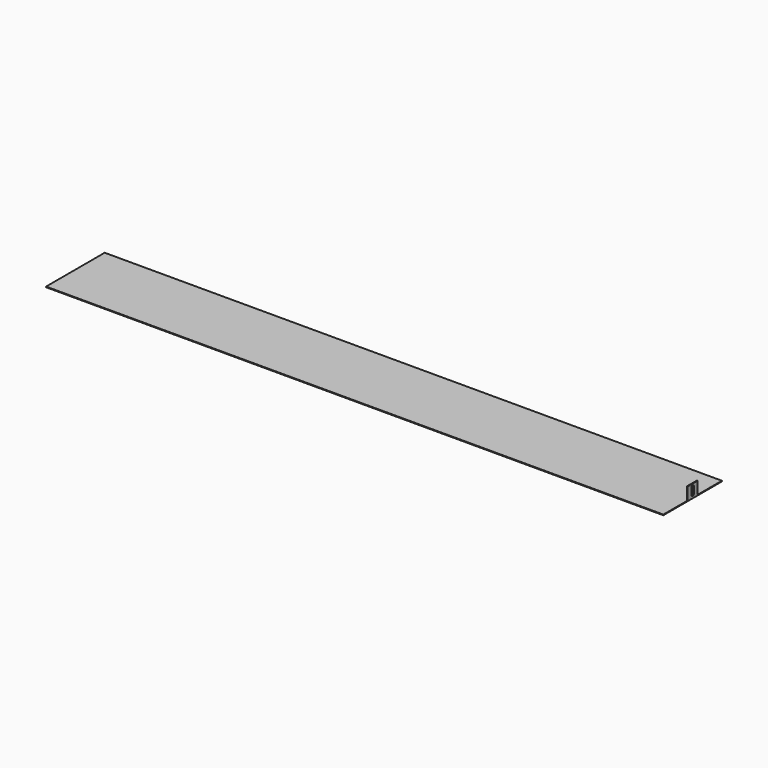
from build123d import *

# Parameters (mm, degrees)
F0_W     = 1500
F0_H     = 178
F1_DEPTH = 1.5875
F2_W     = 30
F2_H     = 30
F3_DEPTH = 1.5875


# Not quite as in the source:
# - a length typed as a fraction of an inch, garbled in the dataset ("3 / 203.2 mm" for 3/8 in), is restored


with BuildPart() as f1:
    # F0 (on Top) → F1 (new body)
    with BuildSketch(Plane.XY):
        with Locations((673.9510029554, 75.5837445271)):
            Rectangle(F0_W, F0_H)
    extrude(amount=F1_DEPTH)

    # F2 (on face) → F3 (join)
    with BuildSketch(Plane.YZ.offset(1423.9510029554)):
        with Locations((75.5837445271, 16.5875)):
            Rectangle(F2_W, F2_H)
        with BuildLine():
            ThreePointArc((71.5837445271, 24.0875), (75.5837445271, 28.0875), (79.5837445271, 24.0875))
            Line((79.5837445271, 24.0875), (79.5837445271, 9.0875))
            ThreePointArc((79.5837445271, 9.0875), (75.5837445271, 5.0875), (71.5837445271, 9.0875))
            Line((71.5837445271, 9.0875), (71.5837445271, 24.0875))
        make_face(mode=Mode.SUBTRACT)
    extrude(amount=-F3_DEPTH)


solid = f1.part
